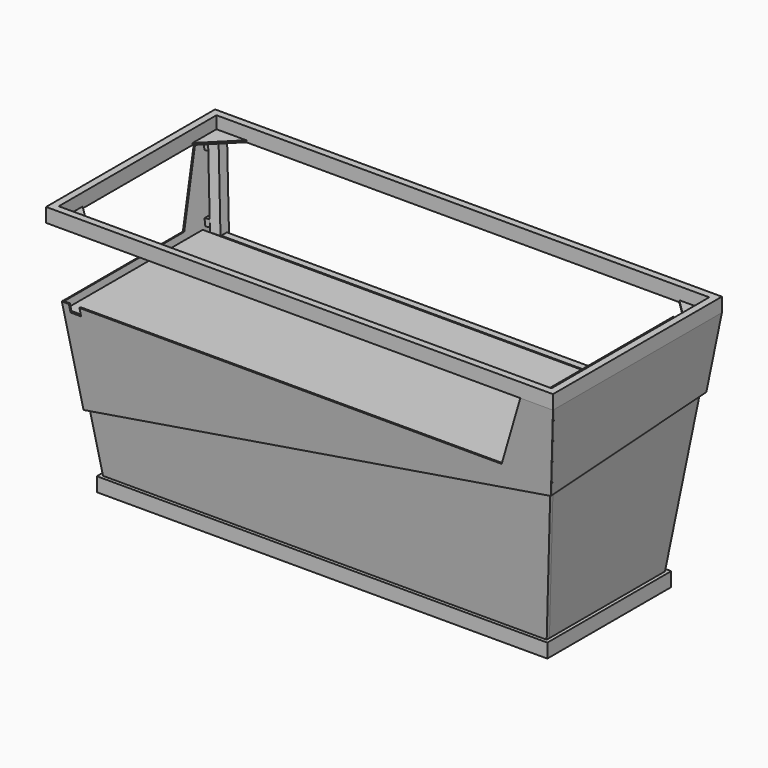
from build123d import *

# Parameters (mm, degrees)
F1_W           = 1828.8
F1_H           = 762
F1_W_2         = 1778
F1_H_2         = 711.2
F2_DEPTH       = 50.8
F3_W           = 1625.6
F3_H           = 558.8
F3_W_2         = 1574.8
F3_H_2         = 508
F4_DEPTH       = 50.8
F7_DEPTH       = 6.35
F11_DEPTH      = 6.35
F16_W          = 38.1
F16_H          = 38.1
F15_W          = 38.1
F15_H          = 38.1
F22_DEPTH      = 4.7625
F25_DEPTH      = 4.7625
F28_DEPTH      = 4.7625
F31_DEPTH      = 12.7
F33_DEPTH      = 12.7
F35_DEPTH      = 12.7
F37_DEPTH      = 116.078
F39_W          = 25.4
F39_H          = 50.8
F40_DEPTH      = 819.912
F40_DEPTH_BACK = 819.912
F42_DEPTH      = 25.4
F45_W          = 25.4
F45_H          = 50.8
F46_DEPTH      = 292.1
F46_DEPTH_BACK = 292.1
F48_DEPTH      = 25.4
F51_DEPTH      = 3.175
F53_DEPTH      = 3.175
F57_DEPTH      = 3.175
F59_DEPTH      = 3.175
F61_DEPTH      = 3.175
F63_DEPTH      = 3.175
F65_W          = 25.4
F65_H          = 25.4
F66_DEPTH      = 20.4413580685
F67_W          = 25.4
F67_H          = 25.4
F68_DEPTH      = 20.4413580685
F69_W          = 25.4
F69_H          = 25.4
F70_DEPTH      = 20.4413580685
F71_W          = 25.4
F71_H          = 25.4
F72_DEPTH      = 20.4413580685
F73_W          = 25.4
F73_H          = 25.4
F74_DEPTH      = 20.4413580685
F75_W          = 25.4
F75_H          = 25.4
F76_DEPTH      = 20.4413580685
F78_W          = 25.4
F78_H          = 25.4
F79_DEPTH      = 20.4413580685
F80_W          = 25.4
F80_H          = 25.4
F81_DEPTH      = 20.4413580685
F83_W          = 25.4
F83_H          = 25.4
F84_DEPTH      = 20.4413580685
F85_W          = 25.4
F85_H          = 25.4
F86_DEPTH      = 20.4413580685
F87_W          = 25.4
F87_H          = 25.4
F88_DEPTH      = 20.4413580685
F89_W          = 25.4
F89_H          = 25.4
F90_DEPTH      = 20.4413580685
F91_W          = 25.4
F91_H          = 50.8
F92_DEPTH      = 819.15
F92_DEPTH_BACK = 819.15
F94_REACH      = 2348.2762927679
F96_REACH      = 952.6286841659


# Not quite as in the source:
# - a feature of the source that left no trace in its solid (it failed there, or was rolled back) is left out
# - a length typed as a fraction of an inch, garbled in the dataset ("3 / 203.2 mm" for 3/8 in), is restored


with BuildPart() as f2:
    # F1 (on offset) → F2 (new body)
    with BuildSketch(Plane.XY.offset(914.4)):
        Rectangle(F1_W, F1_H)
        Rectangle(F1_W_2, F1_H_2, mode=Mode.SUBTRACT)
    extrude(amount=-F2_DEPTH)


with BuildPart() as f4:
    # F3 (on Top) → F4 (new body)
    with BuildSketch(Plane.XY):
        Rectangle(F3_W, F3_H)
        Rectangle(F3_W_2, F3_H_2, mode=Mode.SUBTRACT)
    extrude(amount=F4_DEPTH)


with BuildPart() as f7:
    # F6 (on face) → F7 (new body)
    with BuildSketch(Plane(origin=(0, 0, 863.6), x_dir=(1, 0, 0), z_dir=(0, 0, -1))):
        Polygon((-781.2369265472, 355.6), (-889, 355.6), (-889, 247.8369265472), align=None)
    extrude(amount=-F7_DEPTH)


with BuildPart() as f8_1:
    # F8: instance of F7
    add(f7.part.mirror(Plane.XZ))


with BuildPart() as f9_1:
    # F9: instance of F8_1
    add(f8_1.part.mirror(Plane.YZ))


with BuildPart() as f9_2:
    # F9: instance of F7
    add(f7.part.mirror(Plane.YZ))


with BuildPart() as f11:
    # F10 (on face) → F11 (new body)
    with BuildSketch(Plane.XY.offset(50.8)):
        Polygon((-679.6369265472, 254), (-787.4, 254), (-787.4, 146.2369265472), align=None)
    extrude(amount=-F11_DEPTH)


with BuildPart() as f12_1:
    # F12: instance of F11
    add(f11.part.mirror(Plane.YZ))


with BuildPart() as f13_1:
    # F13: instance of F11
    add(f11.part.mirror(Plane.XZ))


with BuildPart() as f13_2:
    # F13: instance of F12_1
    add(f12_1.part.mirror(Plane.XZ))


with BuildPart() as f17:
    # F16 (on face) → F17 section 0
    with BuildSketch(Plane(origin=(0, 0, 863.6), x_dir=(1, 0, 0), z_dir=(0, 0, -1))):
        with Locations((-869.95, -336.55)):
            Rectangle(F16_W, F16_H)
    # F15 (on face) → F17 section 1
    with BuildSketch(Plane.XY.offset(50.8)):
        with Locations((-768.35, 234.95)):
            Rectangle(F15_W, F15_H)
    loft()


with BuildPart() as f18_1:
    # F18: instance of F17
    add(f17.part.mirror(Plane.XZ))


with BuildPart() as f19_1:
    # F19: instance of F17
    add(f17.part.mirror(Plane.YZ))


with BuildPart() as f19_2:
    # F19: instance of F18_1
    add(f18_1.part.mirror(Plane.YZ))


with BuildPart() as f22:
    # F21 (on 3pt) → F22 (new body)
    with BuildSketch(Plane(origin=(0, -268.8492307692, -33.6061538462), x_dir=(-1, 0, 0), z_dir=(0, 0.9922778767, 0.1240347346))):
        Polygon((839.363427099, 299.2242169315), (882.8951774143, 650.1884082084), (-704.1266299239, 650.1884082084), (-796.5750694275, 904.1884082084), (-914.4, 904.1884082084), (-876.8817135495, 601.70631257), align=None)
    extrude(amount=F22_DEPTH)


with BuildPart() as f25:
    # F24 (on 3pt) → F25 (new body)
    with BuildSketch(Plane(origin=(-794.0430769231, 0, -99.2553846154), x_dir=(0, -1, 0), z_dir=(-0.9922778767, 0, -0.1240347346))):
        Polygon((-289.033561945, 970.3485356383), (-381, 970.3485356383), (-343.4817135495, 667.8664399999), (301.2377037112, 365.9704982076), (344.6967505898, 716.3485356383), (-196.5851224413, 716.3485356383), align=None)
    extrude(amount=-F25_DEPTH)


with BuildPart() as f28:
    # F27 (on 3pt) → F28 (new body)
    with BuildSketch(Plane(origin=(794.0430769231, 0, -99.2553846154), x_dir=(0, -1, 0), z_dir=(-0.9922778767, 0, 0.1240347346))):
        Polygon((338.7559901617, 668.452593846), (376.2015731754, 970.3485356383), (-381, 970.3485356383), (-349.7347612912, 718.2801226063), align=None)
    extrude(amount=F28_DEPTH)


with BuildPart() as f31:
    # F30 (on face) → F31 (new body)
    with BuildSketch(Plane(origin=(0, -243.84, -30.48), x_dir=(1, 0, 0), z_dir=(0, -0.9922778767, -0.1240347346))):
        Polygon((867.6674107563, 625.8738052898), (-830.5433677326, 326.5702017737), (-800.1973194309, 81.9125387227), (800.1973194309, 81.9125387227), align=None)
    extrude(amount=F31_DEPTH)


with BuildPart() as f33:
    # F32 (on face) → F33 (new body)
    with BuildSketch(Plane(origin=(-769.0338461538, 0, -96.1292307692), x_dir=(0, -1, 0), z_dir=(-0.9922778767, 0, -0.1240347346))):
        Polygon((285.4241344213, 401.4221373741), (-334.2100772602, 691.5716952967), (-266.7973194309, 148.0726661526), (254, 148.0726661526), align=None)
    extrude(amount=F33_DEPTH)


with BuildPart() as f35:
    # F34 (on face) → F35 (new body)
    with BuildSketch(Plane(origin=(769.0338461538, 0, -96.1292307692), x_dir=(0, 1, 0), z_dir=(0.9922778767, 0, -0.1240347346))):
        Polygon((340.5995686341, 743.0854216331), (-321.855617202, 695.1421417053), (-254, 148.0726661526), (266.7973194309, 148.0726661526), align=None)
    extrude(amount=F35_DEPTH)


with BuildPart() as f37_tool:
    # F36 (on face) → F37 (new body)
    with BuildSketch(Plane.XZ.offset(381)):
        Polygon((-850.9, 863.6), (-889, 863.6), (-854.075, 584.2), (-815.975, 584.2), align=None)
    extrude(amount=-F37_DEPTH)


with BuildPart() as f18_1_1:
    add(f18_1.part)

    # F37: cut by f37_tool
    add(f37_tool.part, mode=Mode.SUBTRACT)


with BuildPart() as f22_1:
    add(f22.part)

    # F37: cut by f37_tool
    add(f37_tool.part, mode=Mode.SUBTRACT)


with BuildPart() as f40:
    # F39 (on Right) → F40 (new body, two sides)
    with BuildSketch(Plane.YZ) as f40_sk:
        with Locations((-298.45, 558.8)):
            Rectangle(F39_W, F39_H)
    extrude(amount=F40_DEPTH)
    extrude(f40_sk.sketch, amount=-F40_DEPTH_BACK)


with BuildPart() as f42_tool:
    # F41 (on face) → F42 (new body)
    with BuildSketch(Plane.XZ.offset(311.15)):
        Polygon((-809.625, 533.4), (-815.975, 584.2), (-819.912, 584.2), (-819.912, 533.4), align=None)
        Polygon((819.912, 533.4), (819.912, 584.2), (815.975, 584.2), (809.625, 533.4), align=None)
    extrude(amount=-F42_DEPTH)


with BuildPart() as f18_1_2:
    add(f18_1_1.part)

    # F42: cut by f42_tool
    add(f42_tool.part, mode=Mode.SUBTRACT)


with BuildPart() as f19_2_1:
    add(f19_2.part)

    # F42: cut by f42_tool
    add(f42_tool.part, mode=Mode.SUBTRACT)


with BuildPart() as f40_1:
    add(f40.part)

    # F42: cut by f42_tool
    add(f42_tool.part, mode=Mode.SUBTRACT)


with BuildPart() as f43_1:
    # F43: instance of F40
    add(f40_1.part.mirror(Plane.XZ))


with BuildPart() as f46:
    # F45 (on Front) → F46 (new body, two sides)
    with BuildSketch(Plane.XZ) as f46_sk:
        with Locations((-831.85, 558.8)):
            Rectangle(F45_W, F45_H)
    extrude(amount=F46_DEPTH)
    extrude(f46_sk.sketch, amount=-F46_DEPTH_BACK)

    # F47 (on face) → F48 (cut)
    with BuildSketch(Plane(origin=(-844.55, 0, 0), x_dir=(0, -1, 0), z_dir=(-1, 0, 0))):
        Polygon((292.1, 584.2), (282.575, 584.2), (276.225, 533.4), (292.1, 533.4), align=None)
        Polygon((-276.225, 533.4), (-282.575, 584.2), (-292.1, 584.2), (-292.1, 533.4), align=None)
    extrude(amount=-F48_DEPTH, mode=Mode.SUBTRACT)


with BuildPart() as f49_1:
    # F49: instance of F46
    add(f46.part.mirror(Plane.YZ))


with BuildPart() as f51:
    # F50 (on face) → F51 (new body)
    with BuildSketch(Plane(origin=(769.0338461538, 0, -96.1292307692), x_dir=(0, 1, 0), z_dir=(0.9922778767, 0, -0.1240347346))):
        Polygon((187.4693096578, 228.3829758685), (184.3427857869, 203.1761345653), (222.1530477418, 198.486348759), (225.2795716126, 223.6931900622), align=None)
    extrude(amount=-F51_DEPTH)


with BuildPart() as f53:
    # F52 (on face) → F53 (new body)
    with BuildSketch(Plane(origin=(769.0338461538, 0, -96.1292307692), x_dir=(0, 1, 0), z_dir=(0.9922778767, 0, -0.1240347346))):
        Polygon((266.7973251736, 558.4200204013), (269.9238490445, 583.6268617045), (232.1135870897, 588.3166475108), (228.9870632188, 563.1098062076), align=None)
    extrude(amount=-F53_DEPTH)


with BuildPart() as f54_1:
    # F54: instance of F53
    add(f53.part.mirror(Plane.XZ))


with BuildPart() as f54_2:
    # F54: instance of F51
    add(f51.part.mirror(Plane.XZ))


with BuildPart() as f55_1:
    # F55: instance of F54_1
    add(f54_1.part.mirror(Plane.YZ))


with BuildPart() as f55_2:
    # F55: instance of F53
    add(f53.part.mirror(Plane.YZ))


with BuildPart() as f55_3:
    # F55: instance of F51
    add(f51.part.mirror(Plane.YZ))


with BuildPart() as f55_4:
    # F55: instance of F54_2
    add(f54_2.part.mirror(Plane.YZ))


with BuildPart() as f57:
    # F56 (on face) → F57 (new body)
    with BuildSketch(Plane(origin=(0, -243.84, -30.48), x_dir=(1, 0, 0), z_dir=(0, -0.9922778767, -0.1240347346))):
        Polygon((-740.4945306186, 320.446438192), (-778.3047925734, 315.7566523857), (-775.1782687026, 290.5498110825), (-737.3680067478, 295.2395968888), align=None)
    extrude(amount=-F57_DEPTH)


with BuildPart() as f59:
    # F58 (on face) → F59 (new body)
    with BuildSketch(Plane(origin=(0, -243.84, -30.48), x_dir=(1, 0, 0), z_dir=(0, -0.9922778767, -0.1240347346))):
        Polygon((-755.5770061294, 132.5193800259), (-752.4504822586, 107.3125387227), (-714.6402203038, 112.002324529), (-717.7667441746, 137.2091658322), align=None)
    extrude(amount=-F59_DEPTH)


with BuildPart() as f61:
    # F60 (on face) → F61 (new body)
    with BuildSketch(Plane(origin=(0, -243.84, -30.48), x_dir=(1, 0, 0), z_dir=(0, -0.9922778767, -0.1240347346))):
        Polygon((714.6402203038, 112.002324529), (752.4504822586, 107.3125387227), (755.5770061294, 132.5193800259), (717.7667441746, 137.2091658322), align=None)
    extrude(amount=-F61_DEPTH)


with BuildPart() as f63:
    # F62 (on face) → F63 (new body)
    with BuildSketch(Plane(origin=(0, -243.84, -30.48), x_dir=(1, 0, 0), z_dir=(0, -0.9922778767, -0.1240347346))):
        Polygon((800.1, 491.4752323363), (803.2265238709, 516.6820736395), (765.4162619161, 521.3718594458), (762.2897380452, 496.1650181426), align=None)
    extrude(amount=-F63_DEPTH)


with BuildPart() as f66:
    # F65 (on face) → F66 (new body, through all)
    with BuildSketch(Plane(origin=(0, -243.84, -30.48), x_dir=(1, 0, 0), z_dir=(0, -0.9922778767, -0.1240347346))):
        with Locations((865.2242766122, 862.9379259498)):
            Rectangle(F65_W, F65_H)
    extrude(amount=F66_DEPTH)


with BuildPart() as f68:
    # F67 (on face) → F68 (new body, through all)
    with BuildSketch(Plane(origin=(0, -243.84, -30.48), x_dir=(1, 0, 0), z_dir=(0, -0.9922778767, -0.1240347346))):
        with Locations((838.1387565261, 644.5674817697)):
            Rectangle(F67_W, F67_H)
    extrude(amount=F68_DEPTH)


with BuildPart() as f70:
    # F69 (on face) → F70 (new body, through all)
    with BuildSketch(Plane(origin=(0, -243.84, -30.48), x_dir=(1, 0, 0), z_dir=(0, -0.9922778767, -0.1240347346))):
        with Locations((-830.8854304583, 581.3635740905)):
            Rectangle(F69_W, F69_H)
    extrude(amount=F70_DEPTH)


with BuildPart() as f72:
    # F71 (on face) → F72 (new body, through all)
    with BuildSketch(Plane(origin=(0, -243.84, -30.48), x_dir=(1, 0, 0), z_dir=(0, -0.9922778767, -0.1240347346))):
        with Locations((-804.6965759879, 370.2222792177)):
            Rectangle(F71_W, F71_H)
    extrude(amount=F72_DEPTH)


with BuildPart() as f74:
    # F73 (on face) → F74 (new body, through all)
    with BuildSketch(Plane(origin=(-769.0338461538, 0, -96.1292307692), x_dir=(0, -1, 0), z_dir=(-0.9922778767, 0, -0.1240347346))):
        with Locations((297.4854304583, 647.5237015204)):
            Rectangle(F73_W, F73_H)
    extrude(amount=F74_DEPTH)


with BuildPart() as f76:
    # F75 (on face) → F76 (new body, through all)
    with BuildSketch(Plane(origin=(-769.0338461538, 0, -96.1292307692), x_dir=(0, -1, 0), z_dir=(-0.9922778767, 0, -0.1240347346))):
        with Locations((270.986957331, 433.8861812319)):
            Rectangle(F75_W, F75_H)
    extrude(amount=F76_DEPTH)


with BuildPart() as f79:
    # F78 (on face) → F79 (new body, through all)
    with BuildSketch(Plane(origin=(-769.0338461538, 0, -96.1292307692), x_dir=(0, -1, 0), z_dir=(-0.9922778767, 0, -0.1240347346))):
        with Locations((-332.2150458429, 932.2485356383)):
            Rectangle(F78_W, F78_H)
    extrude(amount=F79_DEPTH)


with BuildPart() as f81:
    # F80 (on face) → F81 (new body, through all)
    with BuildSketch(Plane(origin=(-769.0338461538, 0, -96.1292307692), x_dir=(0, -1, 0), z_dir=(-0.9922778767, 0, -0.1240347346))):
        with Locations((-301.7539978027, 709.4631367162)):
            Rectangle(F80_W, F80_H)
    extrude(amount=F81_DEPTH)


with BuildPart() as f84:
    # F83 (on face) → F84 (new body, through all)
    with BuildSketch(Plane(origin=(769.0338461538, 0, -96.1292307692), x_dir=(0, 1, 0), z_dir=(0.9922778767, 0, -0.1240347346))):
        with Locations((331.8242766122, 929.0980533797)):
            Rectangle(F83_W, F83_H)
    extrude(amount=F84_DEPTH)


with BuildPart() as f86:
    # F85 (on face) → F86 (new body, through all)
    with BuildSketch(Plane(origin=(769.0338461538, 0, -96.1292307692), x_dir=(0, 1, 0), z_dir=(0.9922778767, 0, -0.1240347346))):
        with Locations((313.1526491648, 778.5625803186)):
            Rectangle(F85_W, F85_H)
    extrude(amount=F86_DEPTH)


with BuildPart() as f88:
    # F87 (on face) → F88 (new body, through all)
    with BuildSketch(Plane(origin=(769.0338461538, 0, -96.1292307692), x_dir=(0, 1, 0), z_dir=(0.9922778767, 0, -0.1240347346))):
        with Locations((-331.8242766122, 929.0980533797)):
            Rectangle(F87_W, F87_H)
    extrude(amount=F88_DEPTH)


with BuildPart() as f90:
    # F89 (on face) → F90 (new body, through all)
    with BuildSketch(Plane(origin=(769.0338461538, 0, -96.1292307692), x_dir=(0, 1, 0), z_dir=(0.9922778767, 0, -0.1240347346))):
        with Locations((-307.7206870731, 734.7687018569)):
            Rectangle(F89_W, F89_H)
    extrude(amount=F90_DEPTH)


with BuildPart() as f92:
    # F91 (on Right) → F92 (new body, two sides)
    with BuildSketch(Plane.YZ) as f92_sk:
        with Locations((263.525, 558.8)):
            Rectangle(F91_W, F91_H)
    extrude(amount=F92_DEPTH)
    extrude(f92_sk.sketch, amount=-F92_DEPTH_BACK)


with BuildPart() as f94:
    f94_end = Plane(origin=(-109.3530922462, -332.8522073365, 516.8141612179), x_dir=(0, -0.1240347346, 0.9922778767), z_dir=(0, 0.9922778767, 0.1240347346))
    # F93 (on face) → F94 (new body, up to a plane its end follows)
    with BuildSketch(Plane(origin=(0, 276.225, 0), x_dir=(-1, 0, 0), z_dir=(0, 1, 0))):
        Polygon((-815.975, 584.2), (874.6754371842, 584.2), (875.0723121842, 587.375), (-815.975, 587.375), align=None)
    f94_long = extrude(amount=-F94_REACH, mode=Mode.PRIVATE)
    add(split(f94_long, bisect_by=f94_end, keep=Keep.TOP, mode=Mode.PRIVATE))


with BuildPart() as f96:
    f96_end = f22_1.part.faces().sort_by_distance((-109.3530922462, -332.8522073365, 516.8141612179))[0]
    # F95 (on face) → F96 (new body, up to a face of F22 that its end follows)
    with BuildSketch(Plane(origin=(0, 276.225, 0), x_dir=(-1, 0, 0), z_dir=(0, 1, 0))):
        Polygon((-724.7985965885, 587.375), (-721.4167457553, 587.375), (-822.7368298966, 863.6), (-826.1186807298, 863.6), align=None)
    f96_long = extrude(amount=-F96_REACH, mode=Mode.PRIVATE)
    add(split(f96_long, bisect_by=f96_end, keep=Keep.TOP, mode=Mode.PRIVATE))


with BuildPart() as f99_1:
    # F99: copy of F2
    add(f2.part)


solid = Compound([f2.part, f4.part, f7.part, f8_1.part, f9_1.part, f9_2.part, f11.part, f12_1.part, f13_1.part, f13_2.part, f17.part, f19_1.part, f25.part, f28.part, f31.part, f33.part, f35.part, f22_1.part, f18_1_2.part, f19_2_1.part, f40_1.part, f43_1.part, f46.part, f49_1.part, f51.part, f53.part, f54_1.part, f54_2.part, f55_1.part, f55_2.part, f55_3.part, f55_4.part, f57.part, f59.part, f61.part, f63.part, f66.part, f68.part, f70.part, f72.part, f74.part, f76.part, f79.part, f81.part, f84.part, f86.part, f88.part, f90.part, f92.part, f94.part, f96.part, f99_1.part])
